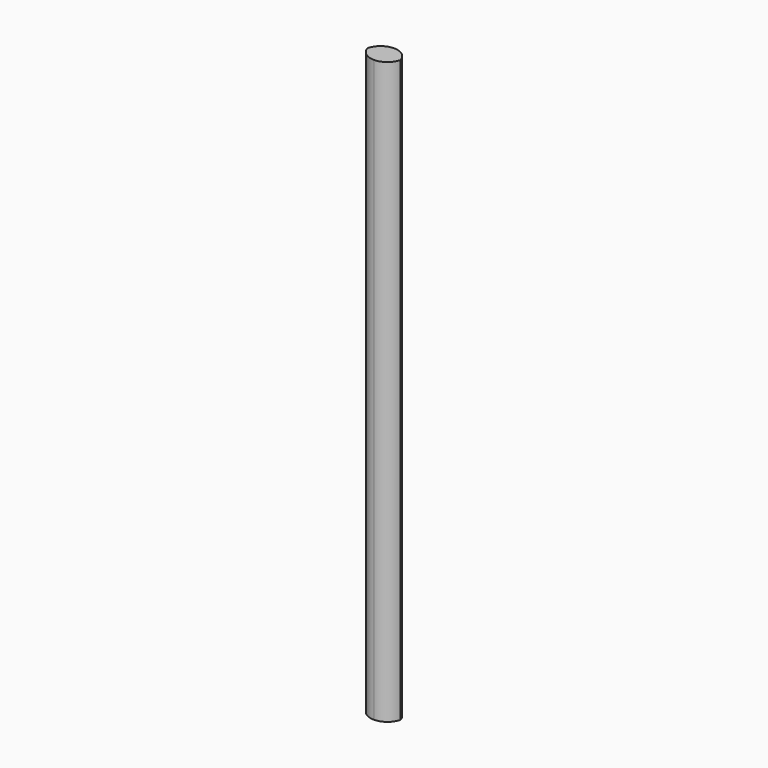
from build123d import *

# Parameters (mm, degrees)
F1_DEPTH    = 7.62
F2_T1_DEPTH = 200.66


# Not quite as in the source:
# - a fillet or chamfer that OpenCascade refuses, or shapes differently, is made with other operations: its cross-section is extruded or revolved along the edge and cut away or added


with BuildPart() as f1:
    # F0 (on Front) → F1 (new body)
    with BuildSketch(Plane.XZ):
        Polygon((10.16, 77.7207358905), (0, 77.7207358905), (0, -72.1392641095), (0, -97.5392641095), (10.16, -97.5392641095), align=None)
    extrude(amount=F1_DEPTH)

    # F2: fillet of radius 5.08 on 4 edges, made by hand

    # F2_s2 → F2_t1 (cut)
    with BuildSketch(Plane.XY.offset(-110.2392641095)):
        with BuildLine():
            ThreePointArc((10.16, -2.54), (8.6721024484, -6.1321024484), (5.08, -7.62))
            Line((5.08, -7.62), (10.16, -7.62))
            Line((10.16, -7.62), (10.16, -2.54))
        make_face()
        with BuildLine():
            ThreePointArc((10.16, -5.08), (8.6721024484, -1.4878975516), (5.08, 0))
            Line((5.08, 0), (10.16, 0))
            Line((10.16, 0), (10.16, -5.08))
        make_face()
        with BuildLine():
            ThreePointArc((5.08, -7.62), (1.4878975516, -6.1321024484), (0, -2.54))
            Line((0, -2.54), (0, -7.62))
            Line((0, -7.62), (5.08, -7.62))
        make_face()
        with BuildLine():
            ThreePointArc((0, -5.08), (1.4878975516, -1.4878975516), (5.08, 0))
            Line((5.08, 0), (0, 0))
            Line((0, 0), (0, -5.08))
        make_face()
    extrude(amount=F2_T1_DEPTH, mode=Mode.SUBTRACT)


solid = f1.part
